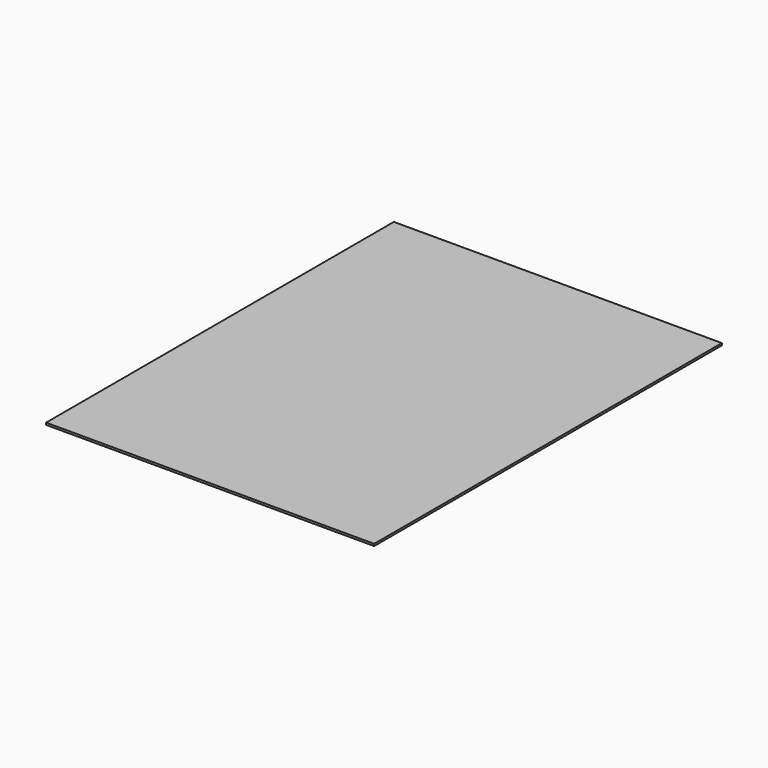
from build123d import *

# Parameters (mm, degrees)
F0_W         = 508
F0_H         = 673.1
F0_TEXT_SIZE = 86.560170394
F1_DEPTH     = 3.175


# Not quite as in the source:
# - Text() gives the source's letters only with a copy of the font that has no kerning and outlines rounded to 1/6400 em; it was checked with that copy


with BuildPart() as f1:
    # F0 (on Top) → F1 (new body)
    with BuildSketch(Plane.XY):
        with Locations((254, -336.55)):
            Rectangle(F0_W, F0_H)
        with BuildLine():
            Line((273.4489882854, -459.7832800852), (273.4489882854, -466.2888178914))
            Line((273.4489882854, -466.2888178914), (232.8333333333, -466.2888178914))
            Line((232.8333333333, -466.2888178914), (232.8333333333, -460.2431309904))
            Line((232.8333333333, -460.2431309904), (249.1039403621, -443.8913738019))
            add(Edge.make_bspline(
                [(249.1039403621, -443.8913738019), (256.5427050053, -436.3579339723), (258.9095846645, -433.1457401491)],
                knots=[0, 0, 0, 1, 1, 1], degree=2))
            add(Edge.make_bspline(
                [(258.9095846645, -433.1457401491), (261.2764643237, -429.9335463259), (262.4599041534, -426.8904153355)],
                knots=[0, 0, 0, 1, 1, 1], degree=2))
            add(Edge.make_bspline(
                [(262.4599041534, -426.8904153355), (263.643343983, -423.847284345), (263.643343983, -420.3443024494)],
                knots=[0, 0, 0, 1, 1, 1], degree=2))
            add(Edge.make_bspline(
                [(263.643343983, -420.3443024494), (263.643343983, -415.394142705), (260.6407880724, -412.4997870075)],
                knots=[0, 0, 0, 1, 1, 1], degree=2))
            add(Edge.make_bspline(
                [(260.6407880724, -412.4997870075), (257.6382321619, -409.6054313099), (252.309371672, -409.6054313099)],
                knots=[0, 0, 0, 1, 1, 1], degree=2))
            add(Edge.make_bspline(
                [(252.309371672, -409.6054313099), (248.4682641108, -409.6054313099), (245.0193823216, -410.8767838126)],
                knots=[0, 0, 0, 1, 1, 1], degree=2))
            add(Edge.make_bspline(
                [(245.0193823216, -410.8767838126), (241.5705005325, -412.1481363152), (237.3506922258, -415.4888178914)],
                knots=[0, 0, 0, 1, 1, 1], degree=2))
            Line((237.3506922258, -415.4888178914), (233.6313099042, -410.7144834931))
            add(Edge.make_bspline(
                [(233.6313099042, -410.7144834931), (242.1656017039, -403.6138445154), (252.2282215122, -403.6138445154)],
                knots=[0, 0, 0, 1, 1, 1], degree=2))
            add(Edge.make_bspline(
                [(252.2282215122, -403.6138445154), (260.9383386581, -403.6138445154), (265.8817358892, -408.0703407881)],
                knots=[0, 0, 0, 1, 1, 1], degree=2))
            add(Edge.make_bspline(
                [(265.8817358892, -408.0703407881), (270.8251331203, -412.5268370607), (270.8251331203, -420.0467518637)],
                knots=[0, 0, 0, 1, 1, 1], degree=2))
            add(Edge.make_bspline(
                [(270.8251331203, -420.0467518637), (270.8251331203, -425.9301384452), (267.5250266241, -431.6782747604)],
                knots=[0, 0, 0, 1, 1, 1], degree=2))
            add(Edge.make_bspline(
                [(267.5250266241, -431.6782747604), (264.2249201278, -437.4264110756), (255.1902023429, -446.2176783813)],
                knots=[0, 0, 0, 1, 1, 1], degree=2))
            Line((255.1902023429, -446.2176783813), (241.6651757188, -459.4451544196))
            Line((241.6651757188, -459.4451544196), (241.6651757188, -459.7832800852))
            Line((241.6651757188, -459.7832800852), (273.4489882854, -459.7832800852))
        make_face(mode=Mode.SUBTRACT)
        Polygon((248.4276890309, -348.5669861555), (240.650798722, -348.5669861555), (266.2536741214, -293.2361022364), (232.5763578275, -293.2361022364), (232.5763578275, -286.7711395101), (273.6924387646, -286.7711395101), (273.6924387646, -292.3975505857), align=None, mode=Mode.SUBTRACT)
        with BuildLine():
            add(Edge.make_bspline(
                [(268.5664536741, -176.2378594249), (273.787113951, -184.4002129925), (273.787113951, -199.8593184239)],
                knots=[0, 0, 0, 1, 1, 1], degree=2))
            add(Edge.make_bspline(
                [(273.787113951, -199.8593184239), (273.787113951, -215.8864749734), (268.7355165069, -223.7918530351)],
                knots=[0, 0, 0, 1, 1, 1], degree=2))
            add(Edge.make_bspline(
                [(268.7355165069, -223.7918530351), (263.6839190628, -231.6972310969), (253.2831735889, -231.6972310969)],
                knots=[0, 0, 0, 1, 1, 1], degree=2))
            add(Edge.make_bspline(
                [(253.2831735889, -231.6972310969), (243.315228967, -231.6972310969), (238.11485623, -223.6025026624)],
                knots=[0, 0, 0, 1, 1, 1], degree=2))
            add(Edge.make_bspline(
                [(238.11485623, -223.6025026624), (232.9144834931, -215.5077742279), (232.9144834931, -199.8593184239)],
                knots=[0, 0, 0, 1, 1, 1], degree=2))
            add(Edge.make_bspline(
                [(232.9144834931, -199.8593184239), (232.9144834931, -183.7239616613), (237.9457933972, -175.8997337593)],
                knots=[0, 0, 0, 1, 1, 1], degree=2))
            add(Edge.make_bspline(
                [(237.9457933972, -175.8997337593), (242.9771033014, -168.0755058573), (253.2831735889, -168.0755058573)],
                knots=[0, 0, 0, 1, 1, 1], degree=2))
            add(Edge.make_bspline(
                [(253.2831735889, -168.0755058573), (263.3457933972, -168.0755058573), (268.5664536741, -176.2378594249)],
                knots=[0, 0, 0, 1, 1, 1], degree=2))
        make_face(mode=Mode.SUBTRACT)
        with BuildLine():
            Line((258.8149094782, -51.3274760383), (258.8149094782, -113.1233226837))
            Line((258.8149094782, -113.1233226837), (251.9712460064, -113.1233226837))
            Line((251.9712460064, -113.1233226837), (251.9712460064, -69.0858359957))
            add(Edge.make_bspline(
                [(251.9712460064, -69.0858359957), (251.9712460064, -63.5811501597), (252.309371672, -58.6850905218)],
                knots=[0, 0, 0, 1, 1, 1], degree=2))
            add(Edge.make_bspline(
                [(252.309371672, -58.6850905218), (251.4302449414, -59.577742279), (250.3279552716, -60.5447816826)],
                knots=[0, 0, 0, 1, 1, 1], degree=2))
            add(Edge.make_bspline(
                [(250.3279552716, -60.5447816826), (249.2256656017, -61.5118210863), (240.2720979766, -68.78828541)],
                knots=[0, 0, 0, 1, 1, 1], degree=2))
            Line((240.2720979766, -68.78828541), (236.552715655, -63.9733759318))
            Line((236.552715655, -63.9733759318), (252.9044728435, -51.3274760383))
            Line((252.9044728435, -51.3274760383), (258.8149094782, -51.3274760383))
        make_face(mode=Mode.SUBTRACT)
        with Locations((228.6, -230.8451544196)):
            Text('0', F0_TEXT_SIZE, font='Open Sans', text_align=(TextAlign.LEFT, TextAlign.BOTTOM))
        with BuildLine():
            add(Edge.make_bspline(
                [(243.1867412141, -180.2683173589), (240.0151224707, -186.3748668797), (240.0151224707, -199.8593184239)],
                knots=[0, 0, 0, 1, 1, 1], degree=2))
            add(Edge.make_bspline(
                [(240.0151224707, -199.8593184239), (240.0151224707, -213.3437699681), (243.1867412141, -219.497657082)],
                knots=[0, 0, 0, 1, 1, 1], degree=2))
            add(Edge.make_bspline(
                [(243.1867412141, -219.497657082), (246.3583599574, -225.651544196), (253.2831735889, -225.651544196)],
                knots=[0, 0, 0, 1, 1, 1], degree=2))
            add(Edge.make_bspline(
                [(253.2831735889, -225.651544196), (260.3026624068, -225.651544196), (263.4472310969, -219.4165069223)],
                knots=[0, 0, 0, 1, 1, 1], degree=2))
            add(Edge.make_bspline(
                [(263.4472310969, -219.4165069223), (266.591799787, -213.1814696486), (266.591799787, -199.8593184239)],
                knots=[0, 0, 0, 1, 1, 1], degree=2))
            add(Edge.make_bspline(
                [(266.591799787, -199.8593184239), (266.591799787, -186.5506922258), (263.4472310969, -180.3562300319)],
                knots=[0, 0, 0, 1, 1, 1], degree=2))
            add(Edge.make_bspline(
                [(263.4472310969, -180.3562300319), (260.3026624068, -174.1617678381), (253.2831735889, -174.1617678381)],
                knots=[0, 0, 0, 1, 1, 1], degree=2))
            add(Edge.make_bspline(
                [(253.2831735889, -174.1617678381), (246.3583599574, -174.1617678381), (243.1867412141, -180.2683173589)],
                knots=[0, 0, 0, 1, 1, 1], degree=2))
        make_face()
        with Locations((228.6, -113.1233226837)):
            Text('1', F0_TEXT_SIZE, font='Open Sans', text_align=(TextAlign.LEFT, TextAlign.BOTTOM))
        with Locations((228.6, -466.2888178914)):
            Text('2', F0_TEXT_SIZE, font='Open Sans', text_align=(TextAlign.LEFT, TextAlign.BOTTOM))
        with Locations((228.6, -348.5669861555)):
            Text('7', F0_TEXT_SIZE, font='Open Sans', text_align=(TextAlign.LEFT, TextAlign.BOTTOM))
    extrude(amount=F1_DEPTH)


solid = f1.part
